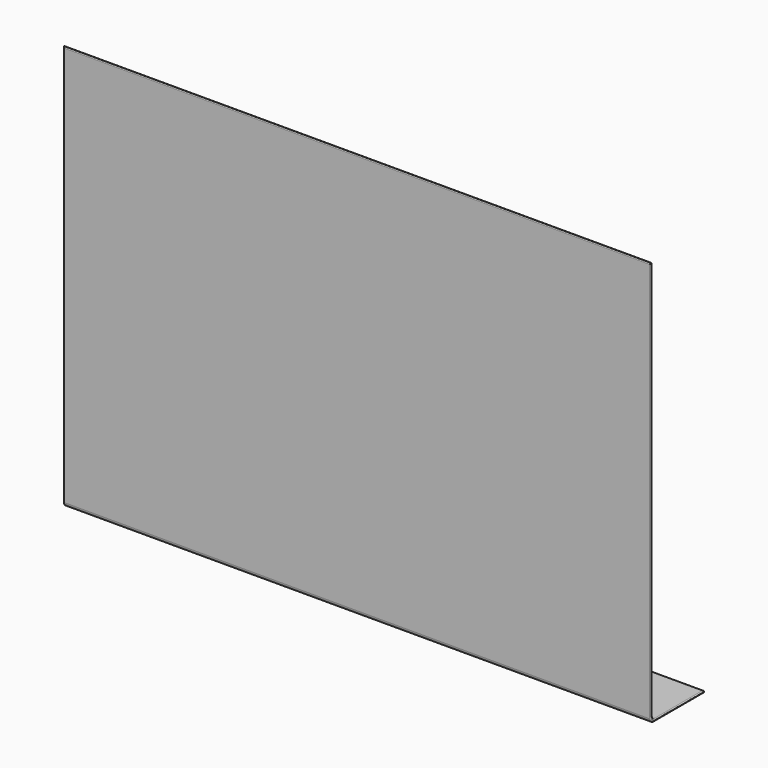
from build123d import *

# Parameters (mm, degrees)
F2_DEPTH = 261
F3_R     = 3.6
F4_R     = 0.89999


# Not quite as in the source:
# - a fillet or chamfer is up to 0.001 mm smaller than in the source, because OpenCascade refuses the exact size


with BuildPart() as f2:
    # F1 (on Right) → F2 (new body)
    with BuildSketch(Plane.YZ):
        Polygon((0, 360), (0, 0), (59.5, 0), (59.5, 1.8), (1.8, 1.8), (1.8, 360), align=None)
    extrude(amount=F2_DEPTH)

    # F3
    f3_edges = [f2.edges().sort_by_distance(p)[0] for p in [
        (130.5, 1.8, 1.8),
        (130.5, 0, 0),
    ]]
    fillet(f3_edges, radius=F3_R)

    # F4 (radius 0.9 in the source; OpenCascade refuses exactly that, so slightly less here)
    f4_edges = [f2.edges().sort_by_distance(p)[0] for p in [
        (261, 32.45, 1.8),
        (261, 31.55, 0),
        (130.5, 59.5, 1.8),
        (130.5, 59.5, 0),
        (261, 1.8, 182.7),
        (261, 0, 181.8),
        (130.5, 0, 360),
        (130.5, 1.8, 360),
        (261, 1.054416, 1.054416),
    ]]
    fillet(f4_edges, radius=F4_R)

    # F5: F2 across face


with BuildPart() as f2_1:
    add(f2.part)
    add(f2.part.mirror(Plane(origin=(0, 4.9930290886, 155.2430290886), x_dir=(0, 1, 0), z_dir=(-1, 0, 0))))


solid = f2_1.part
